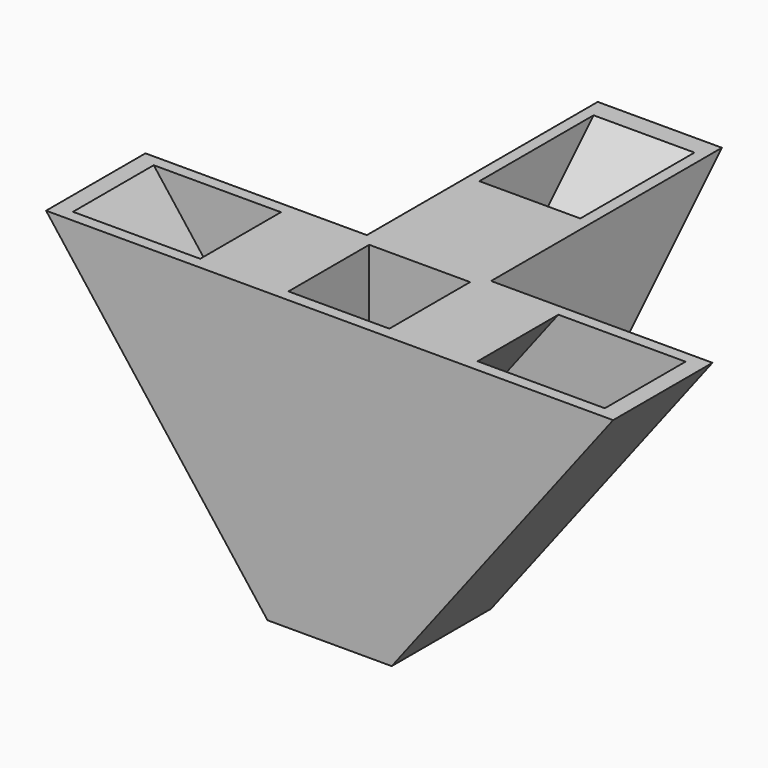
from build123d import *

# Parameters (mm, degrees)
F1_DEPTH      = 16
F3_DEPTH      = 8
F3_DEPTH_BACK = 8
F4_W          = 16
F4_H          = 10.4258029827
F5_DEPTH      = 45.4
F7_DEPTH      = 25
F9_START      = -1.5
F9_DEPTH      = 13
F11_START     = -1.5
F11_DEPTH     = 13
F12_W         = 13
F12_H         = 13
F13_DEPTH     = 45.8


# Not quite as in the source:
# - a feature of the source that left no trace in its solid (it failed there, or was rolled back) is left out


with BuildPart() as f1:
    # F0 (on Front) → F1 (new body)
    with BuildSketch(Plane.XZ):
        Polygon((-36.5256857405, 47.6012004175), (0, 0), (36.5256857405, 47.6012004175), align=None)
    extrude(amount=F1_DEPTH)

    # F2 (on Right) → F3 (join, two sides)
    with BuildSketch(Plane.YZ) as f3_sk:
        Polygon((0, 47.6012004175), (0, 0), (47.6012004175, 47.6012004175), align=None)
    extrude(amount=F3_DEPTH)
    extrude(f3_sk.sketch, amount=-F3_DEPTH_BACK)

    # F4 (on face) → F5 (cut)
    with BuildSketch(Plane.XZ.offset(16)):
        with Locations((0, 5.2129014914)):
            Rectangle(F4_W, F4_H)
    extrude(amount=-F5_DEPTH, mode=Mode.SUBTRACT)

    # F6 (on face) → F7 (cut)
    with BuildSketch(Plane.YZ.offset(8)):
        Polygon((37.1753974347, 47.6012004175), (0, 10.4258029827), (10.4258029827, 10.4258029827), (47.6012004175, 47.6012004175), align=None)
    extrude(amount=-F7_DEPTH, mode=Mode.SUBTRACT)

    # F8 (on face) → F9 (cut)
    with BuildSketch(Plane.XZ.offset(16).offset(F9_START)):
        Polygon((-54.3261755364, 73.7560737056), (-17.2410544745, 25.4258029827), (-6.9274610507, 33.3397015598), (-44.0125821126, 81.6699722827), align=None)
        Polygon((6.9274610507, 33.3397015598), (17.2410544745, 25.4258029827), (53.1179434037, 72.181474934), (42.8043499799, 80.0953735111), align=None)
    extrude(amount=-F9_DEPTH, mode=Mode.SUBTRACT)

    # F10 (on face) → F11 (cut)
    with BuildSketch(Plane(origin=(-8, 0, 0), x_dir=(0, -1, 0), z_dir=(-1, 0, 0)).offset(F11_START)):
        Polygon((-16.2450367116, 47.6012004175), (-34.6298130225, 47.6012004175), (-9.8810756809, 22.8524630759), (-0.6886875255, 32.0448512314), align=None)
    extrude(amount=-F11_DEPTH, mode=Mode.SUBTRACT)

    # F12 (on face) → F13 (cut)
    with BuildSketch(Plane(origin=(0, 0, 10.4258029827), x_dir=(1, 0, 0), z_dir=(0, 0, -1))):
        with Locations((0, 8)):
            Rectangle(F12_W, F12_H)
    extrude(amount=-F13_DEPTH, mode=Mode.SUBTRACT)


solid = f1.part
